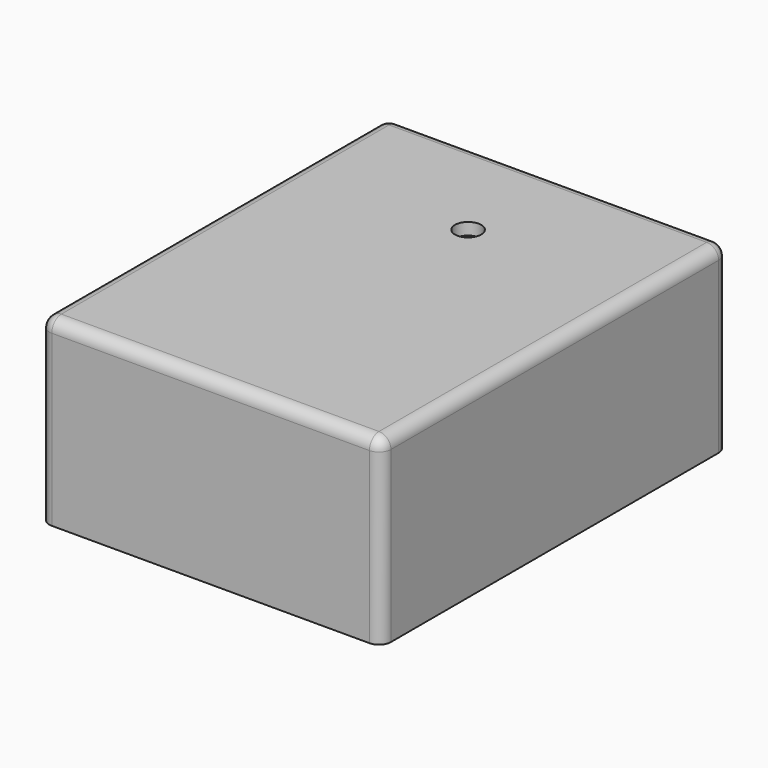
from build123d import *

# Parameters (mm, degrees)
F3_W     = 14.3
F3_H     = 18.15
F4_DEPTH = 7.6
F5_R     = 0.5
F0_T     = 0.5
F2_D     = 1.1


# Not quite as in the source:
# - a shell that OpenCascade refuses in one call is made with other operations: the cavity is built on its own and cut out


with BuildPart() as f4:
    # F3 (on Top) → F4 (new body)
    with BuildSketch(Plane.XY):
        Rectangle(F3_W, F3_H)
    extrude(amount=F4_DEPTH)

    # F5
    f5_edges = [f4.edges().sort_by_distance(p)[0] for p in [
        (-7.15, -9.075, 3.8),
        (7.15, -9.075, 3.8),
        (7.15, 0, 7.6),
        (-7.15, 9.075, 3.8),
        (7.15, 9.075, 3.8),
        (-7.15, 0, 7.6),
        (0, 9.075, 7.6),
        (0, -9.075, 7.6),
    ]]
    fillet(f5_edges, radius=F5_R)

    # F0: shell of thickness 0.5, made by hand


with BuildPart() as f0_core1:
    # F0_t2: copy of F4
    add(f4.part)

    # the walls: a layer under each face that stays
    f0_faces = [f0_core1.faces().sort_by_distance(p)[0] for p in [
        (0, -9.075, 3.55),
        (-7.15, 0, 3.55),
        (7.15, 0, 3.55),
        (0, 9.075, 3.55),
        (0, 0, 7.6),
    ]]
    thicken(f0_faces, amount=-F0_T, mode=Mode.SUBTRACT)


with BuildPart() as f4_1:
    add(f4.part)

    # what is left inside the walls is the cavity
    f0_cavity = [f0_core1.part.solids().sort_by_distance(p)[0] for p in [
        (0, -2.858333, 0.005),
    ]]
    add(f0_cavity, mode=Mode.SUBTRACT)

    # F2 (through all)
    with Locations(Plane.XY.offset(7.6)):
        with Locations((0, 4.4)):
            Hole(F2_D / 2)


solid = f4_1.part
